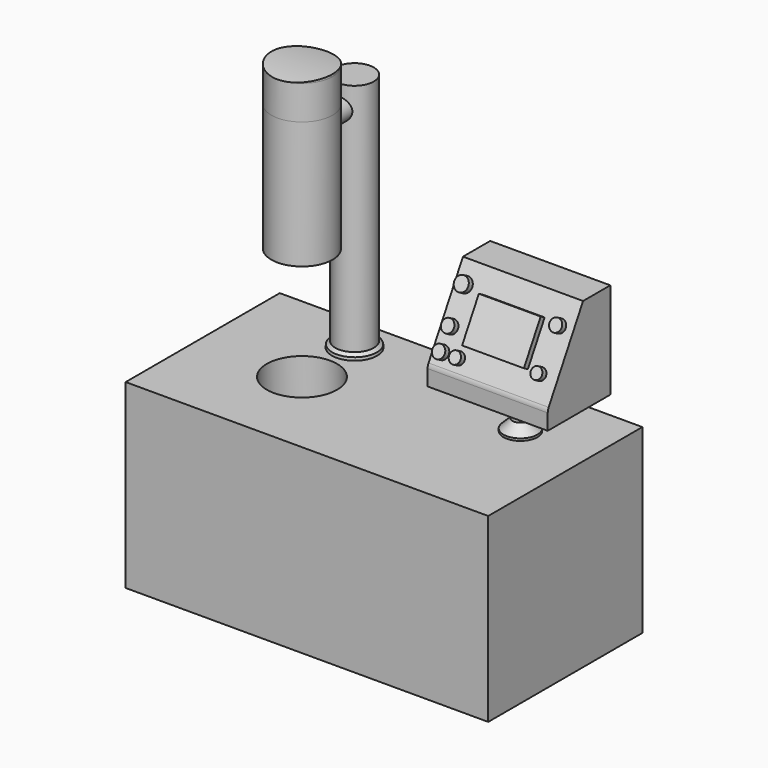
from build123d import *
from build123d import SkipClean  # not in build123d's __all__

# Parameters (mm, degrees)
F0_W      = 1600
F0_H      = 850
F1_DEPTH  = 800
F2_R      = 155
F3_DEPTH  = 210
F4_R      = 100
F5_DEPTH  = 25.4
F5_TAPER  = 6
F7_R      = 84.6303524243
F8_DEPTH  = 1034.6
F9_R      = 75
F10_DEPTH = 50
F11_SIZE  = 40
F12_R     = 35
F13_DEPTH = 100
F14_R     = 100
F15_DEPTH = 10
F18_DEPTH = 265
F20_R     = 50
F21_DEPTH = 150
F22_R     = 134.9695088885
F22_R_2   = 131.9695088885
F23_DEPTH = 561.34
F24_R     = 134.9695088885
F24_R_2   = 131.9695088885
F25_DEPTH = 150
F28_DEPTH = 134.747
F30_DEPTH = 25.4
F32_DEPTH = 25.4
F34_DEPTH = 25.4
F36_DEPTH = 25.4
F37_R     = 31.0271964064
F37_R_2   = 27.8958895213
F37_R_3   = 27.5153110401
F37_R_4   = 25.3697871684
F37_R_5   = 27.0215738096
F37_R_6   = 24.8073241301
F37_W     = 272.6435363293
F37_H     = 187.8117322922
F38_DEPTH = 25.4


# Not quite as in the source:
# - a fillet or chamfer that OpenCascade refuses, or shapes differently, is made with other operations: its cross-section is extruded or revolved along the edge and cut away or added


with BuildPart() as f1:
    # F0 (on Top) → F1 (new body)
    with BuildSketch(Plane.XY):
        Rectangle(F0_W, F0_H)
    extrude(amount=-F1_DEPTH)

    # F2 (on face) → F3 (cut)
    with BuildSketch(Plane.XY):
        with Locations((-350, -15)):
            Circle(F2_R)
    extrude(amount=-F3_DEPTH, mode=Mode.SUBTRACT)

    # F4 (on face) → F5 (join)
    with BuildSketch(Plane.XY):
        with Locations((-345.8311867569, 269.9695088885)):
            Circle(F4_R)
    extrude(amount=F5_DEPTH, taper=F5_TAPER)

    # F6: chamfer of 12.7 on 1 edges, made by hand

    # F6_s1 → F6_t2 (revolve, cut)
    with BuildSketch(Plane.XZ.offset(-269.9695088885)):
        Polygon((-247.1733228492, 12.7695719288), (-261.2008343327, 25.4), (-248.5008343327, 25.4), align=None)
    revolve(axis=Axis((-345.8311867569, 269.9695088885, 25.4), (0, 0, -1)), mode=Mode.SUBTRACT)

    # F7 (on face) → F8 (join)
    with BuildSketch(Plane.XY.offset(25.4)):
        with Locations((-345.8311867569, 269.9695088885)):
            Circle(F7_R)
    extrude(amount=F8_DEPTH)

    # F9 (on face) → F10 (join)
    with BuildSketch(Plane.XY):
        with Locations((490, 140)):
            Circle(F9_R)
    extrude(amount=F10_DEPTH)

    # F11
    f11_edges = [f1.edges().sort_by_distance(p)[0] for p in [
        (415, 140, 50),
    ]]
    chamfer(f11_edges, length=F11_SIZE)

    # F12 (on face) → F13 (join)
    with BuildSketch(Plane.XY.offset(50)):
        with Locations((490, 140)):
            Circle(F12_R)
    extrude(amount=F13_DEPTH)

    # F14 (on face) → F15 (join)
    with BuildSketch(Plane.XY.offset(150)):
        with Locations((490, 140)):
            Circle(F14_R)
    extrude(amount=F15_DEPTH)

    # F17 (on face) → F18 (join, symmetric)
    with BuildSketch(Plane.YZ.offset(490)):
        with BuildLine():
            Line((304.3540355563, 585), (154.3540355563, 585))
            Line((154.3540355563, 585), (-35.4684779925, 249.1601683367))
            ThreePointArc((-35.4684779925, 249.1601683367), (-39.3299439569, 239.6538167994), (-40.6459644437, 229.47787807))
            Line((-40.6459644437, 229.47787807), (-40.6459644437, 160))
            Line((-40.6459644437, 160), (304.3540355563, 160))
            Line((304.3540355563, 160), (304.3540355563, 585))
        make_face()
    extrude(amount=F18_DEPTH, both=True)

    # F20 (on face) → F21 (join)
    with BuildSketch(Plane(origin=(0, 269.9695088885, 0), x_dir=(-1, 0, 0), z_dir=(0, 1, 0))):
        with Locations((349.1199016571, 960)):
            Circle(F20_R)
    extrude(amount=-F21_DEPTH)

    # F37 (on face) → F38 (join)
    with BuildSketch(Plane(origin=(0, -133.6127724795, 75.5202627058), x_dir=(1, 0, 0), z_dir=(0, -0.8705628387, 0.4920572567))):
        with Locations((269.7143256664, 497.251868248)):
            Circle(F37_R)
        with Locations((269.7143256664, 344.7649217223)):
            Circle(F37_R_2)
        with Locations((266.8685615063, 250.4745423794)):
            Circle(F37_R_3)
        with Locations((338.7044257195, 250.4745423794)):
            Circle(F37_R_4)
        with Locations((694.3796277046, 476.1908352375)):
            Circle(F37_R_5)
        with Locations((679.8734068871, 297.5423932076)):
            Circle(F37_R_6)
        with Locations((488.1581813097, 392.0264542103)):
            Rectangle(F37_W, F37_H)
    extrude(amount=F38_DEPTH)


with BuildPart() as f23:
    # F22 (on face) → F23 (new body)
    with BuildSketch(Plane.XY.offset(1060)):
        with Locations((-350, -15)):
            Circle(F22_R)
        with Locations((-350, -15)):
            Circle(F22_R_2, mode=Mode.SUBTRACT)
    extrude(amount=-F23_DEPTH)

    # F24 (on face) → F25 (join)
    with BuildSketch(Plane.XY.offset(1060)):
        with Locations((-350, -15)):
            Circle(F24_R)
        with Locations((-350, -15)):
            Circle(F24_R_2, mode=Mode.SUBTRACT)
    extrude(amount=F25_DEPTH)

    # F27 (on face) → F28 (join, symmetric)
    with BuildSketch(Plane.YZ.offset(-350)):
        with BuildLine():
            Line((-149.7469991446, 1210), (119.3135008216, 1210))
            ThreePointArc((119.3135008216, 1210), (-15.2167491615, 1220), (-149.7469991446, 1210))
        make_face()
    extrude(amount=F28_DEPTH, both=True)

    # F29 (on face) → F30 (cut)
    with BuildSketch(Plane(origin=(0, 0, 1210), x_dir=(1, 0, 0), z_dir=(0, 0, -1))):
        with BuildLine():
            Line((-484.747, 7.2531089721), (-484.747, -119.3135008216))
            Line((-484.747, -119.3135008216), (-363.2910430985, -119.3135008216))
            ThreePointArc((-363.2910430985, -119.3135008216), (-447.3837369881, -78.451463872), (-484.747, 7.2531089721))
        make_face()
    extrude(amount=-F30_DEPTH, mode=Mode.SUBTRACT)

    # F31 (on face) → F32 (cut)
    with BuildSketch(Plane(origin=(0, 0, 1210), x_dir=(1, 0, 0), z_dir=(0, 0, -1))):
        with BuildLine():
            Line((-357.7469059073, 149.7469991446), (-484.747, 149.7469991446))
            Line((-484.747, 149.7469991446), (-484.747, 22.7468910279))
            ThreePointArc((-484.747, 22.7468910279), (-445.4378602578, 110.4378497191), (-357.7469059073, 149.7469991446))
        make_face()
    extrude(amount=-F32_DEPTH, mode=Mode.SUBTRACT)

    # F33 (on face) → F34 (cut)
    with BuildSketch(Plane(origin=(0, 0, 1210), x_dir=(1, 0, 0), z_dir=(0, 0, -1))):
        with BuildLine():
            Line((-336.7089569015, -119.3135008216), (-215.253, -119.3135008216))
            Line((-215.253, -119.3135008216), (-215.253, 7.2531089721))
            ThreePointArc((-215.253, 7.2531089721), (-252.6162630119, -78.451463872), (-336.7089569015, -119.3135008216))
        make_face()
    extrude(amount=-F34_DEPTH, mode=Mode.SUBTRACT)

    # F35 (on face) → F36 (cut)
    with BuildSketch(Plane(origin=(0, 0, 1210), x_dir=(1, 0, 0), z_dir=(0, 0, -1))):
        with BuildLine():
            Line((-215.253, 22.7468910279), (-215.253, 149.7469991446))
            Line((-215.253, 149.7469991446), (-342.2530940927, 149.7469991446))
            ThreePointArc((-342.2530940927, 149.7469991446), (-254.5621397422, 110.4378497191), (-215.253, 22.7468910279))
        make_face()
    with SkipClean():  # cleaning this boolean's faces spoils the solid; the shape is the same uncleaned
        extrude(amount=-F36_DEPTH, mode=Mode.SUBTRACT)


solid = Compound([f1.part, f23.part])
